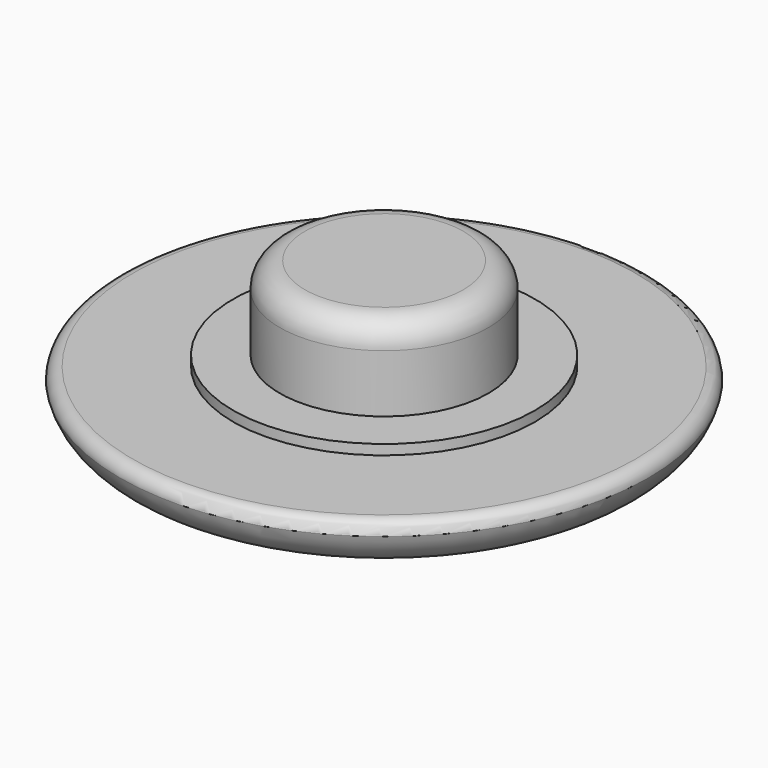
from build123d import *

# Parameters (mm, degrees)
F0_R     = 10.5
F0_R_2   = 6
F1_DEPTH = 2
F0_R_3   = 4.15
F2_DEPTH = 2.4
F3_DEPTH = 5.7
F4_R     = 1
F5_R     = 0.5
F7_R     = 7
F7_R_2   = 6.5
F7_R_3   = 6
F7_R_4   = 5
F7_R_5   = 4.5
F7_R_6   = 4.15
F7_R_7   = 4
F7_R_8   = 3
F7_R_9   = 2.5
F7_R_10  = 2
F7_R_11  = 1
F7_R_12  = 0.5
F8_DEPTH = 1
F9_R     = 0.49999
F10_R    = 0.49999


# Not quite as in the source:
# - a fillet or chamfer that OpenCascade refuses, or shapes differently, is made with other operations: its cross-section is extruded or revolved along the edge and cut away or added
# - a fillet or chamfer is up to 0.001 mm smaller than in the source, because OpenCascade refuses the exact size


with BuildPart() as f1:
    # F0 (on Top) → F1 (new body)
    with BuildSketch(Plane.XY):
        Circle(F0_R)
        Circle(F0_R_2, mode=Mode.SUBTRACT)
    extrude(amount=F1_DEPTH)

    # F0 (on Top) → F2 (join)
    with BuildSketch(Plane.XY):
        Circle(F0_R_2)
        Circle(F0_R_3, mode=Mode.SUBTRACT)
    extrude(amount=F2_DEPTH)

    # F0 (on Top) → F3 (join)
    with BuildSketch(Plane.XY):
        Circle(F0_R_3)
    extrude(amount=F3_DEPTH)

    # F4
    f4_edges = [f1.edges().sort_by_distance(p)[0] for p in [
        (-4.15, 0, 5.7),
    ]]
    fillet(f4_edges, radius=F4_R)

    # F5
    f5_edges = [f1.edges().sort_by_distance(p)[0] for p in [
        (-10.5, 0, 2),
    ]]
    fillet(f5_edges, radius=F5_R)

    # F6: fillet of radius 2 on 1 edges, made by hand

    # F6_s1 → F6_t2 (revolve, cut)
    with BuildSketch(Plane.XZ):
        with BuildLine():
            ThreePointArc((10.5, 1.5), (9.7882531983, 0.4188611699), (8.5635083269, 0))
            Line((8.5635083269, 0), (8.5635083269, -0.04))
            Line((8.5635083269, -0.04), (10.5, -0.04))
            Line((10.5, -0.04), (10.54, 0))
            ThreePointArc((10.54, 0), (10.54, 0.75), (10.5387298335, 1.49))
            Line((10.5387298335, 1.49), (10.5, 1.5))
        make_face()
    revolve(axis=Axis((0, 0, 0), (0, 0, 1)), mode=Mode.SUBTRACT)

    # F7 (on face) → F8 (cut)
    with BuildSketch(Plane.XY):
        Circle(F7_R)
        Circle(F7_R_2, mode=Mode.SUBTRACT)
        Circle(F7_R_2)
        Circle(F7_R_3, mode=Mode.SUBTRACT)
        Circle(F7_R_4)
        Circle(F7_R_5, mode=Mode.SUBTRACT)
        Circle(F7_R_5)
        Circle(F7_R_6, mode=Mode.SUBTRACT)
        Circle(F7_R_6)
        Circle(F7_R_7, mode=Mode.SUBTRACT)
        Circle(F7_R_8)
        Circle(F7_R_9, mode=Mode.SUBTRACT)
        Circle(F7_R_9)
        Circle(F7_R_10, mode=Mode.SUBTRACT)
        Circle(F7_R_11)
        Circle(F7_R_12, mode=Mode.SUBTRACT)
        Circle(F7_R_12)
    extrude(amount=F8_DEPTH, mode=Mode.SUBTRACT)

    # F9 (radius 0.5 in the source; OpenCascade refuses exactly that, so slightly less here)
    f9_edges = [f1.edges().sort_by_distance(p)[0] for p in [
        (-1, 0, 0),
        (-2, 0, 0),
        (-3, 0, 0),
        (-4, 0, 0),
        (-6, 0, 0),
        (-5, 0, 0),
        (-7, 0, 0),
    ]]
    fillet(f9_edges, radius=F9_R)

    # F10 (radius 0.5 in the source; OpenCascade refuses exactly that, so slightly less here)
    f10_edges = [f1.edges().sort_by_distance(p)[0] for p in [
        (-6, 0, 1),
        (-7, 0, 1),
        (-4, 0, 1),
        (-5, 0, 1),
        (-2, 0, 1),
        (-3, 0, 1),
        (-1, 0, 1),
    ]]
    fillet(f10_edges, radius=F10_R)


solid = f1.part
